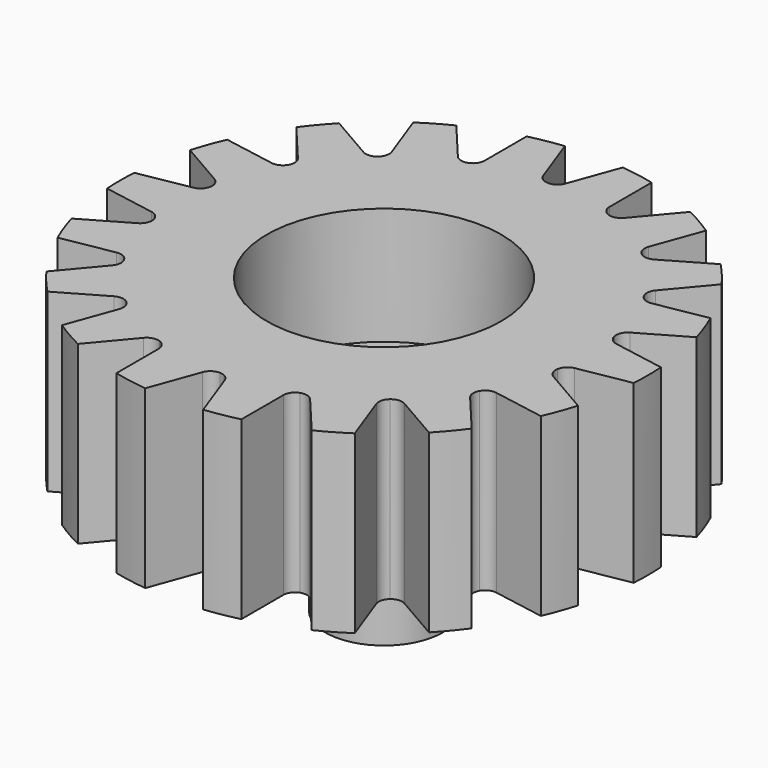
from build123d import *

# Parameters (mm, degrees)
F0_R            = 10
F0_R_2          = 5
F1_DEPTH        = 5
F2_DEPTH        = 15
F3_R            = 2
F4_DEPTH        = 8.6998377653
F0_R_3          = 22.5
F0_R_4          = 17.5
F5_DEPTH        = 5
F6_DEPTH        = 10
F8_DEPTH        = 25.0010001
F8_COPIES_COUNT = 18


# Not quite as in the source:
# - a feature of the source that left no trace in its solid (it failed there, or was rolled back) is left out
# - a pattern or mirror of a feature is missing from the dataset's text; its kind, count and spacing are read off the source's solid


with BuildPart() as f1:
    # F0 (on Top) → F1 (new body)
    with BuildSketch(Plane.XY):
        Circle(F0_R)
        Circle(F0_R_2, mode=Mode.SUBTRACT)
    extrude(amount=-F1_DEPTH)

    # F0 (on Top) → F2 (join)
    with BuildSketch(Plane.XY):
        Circle(F0_R_2)
        with BuildLine():
            ThreePointArc((2.1347076706, 1.3011622347), (2.4069450738, 0.6757332401), (2.5, 0))
            ThreePointArc((2.5, 0), (-0.6757332401, -2.4069450738), (-2.1347076706, 1.3011622347))
            ThreePointArc((-2.1347076706, 1.3011622347), (0, 2.5), (2.1347076706, 1.3011622347))
        make_face(mode=Mode.SUBTRACT)
        with BuildLine():
            Line((-2.1347076706, 1.3011622347), (2.1347076706, 1.3011622347))
            ThreePointArc((2.1347076706, 1.3011622347), (0, 2.5), (-2.1347076706, 1.3011622347))
        make_face()
    extrude(amount=-F2_DEPTH)

    # F3 (on face) → F4 (cut, through all)
    with BuildSketch(Plane.XZ.offset(-1.3011622347)):
        with Locations((0, -10)):
            Circle(F3_R)
    extrude(amount=-F4_DEPTH, mode=Mode.SUBTRACT)

    # F0 (on Top) → F5 (join)
    with BuildSketch(Plane.XY):
        Circle(F0_R_3)
        Circle(F0_R_4, mode=Mode.SUBTRACT)
        Circle(F0_R_4)
        Circle(F0_R, mode=Mode.SUBTRACT)
    extrude(amount=-F5_DEPTH)

    # F0 (on Top) → F6 (join)
    with BuildSketch(Plane.XY):
        Circle(F0_R_3)
        Circle(F0_R_4, mode=Mode.SUBTRACT)
        Circle(F0_R_4)
        Circle(F0_R, mode=Mode.SUBTRACT)
    extrude(amount=F6_DEPTH)

    # F7 (on face) → F8 (cut, through all)
    with BuildSketch(Plane.XY.offset(10)):
        with BuildLine():
            Line((0.9396926208, 18.1579798567), (2.470541887, 22.3639536483))
            ThreePointArc((2.470541887, 22.3639536483), (0, 22.5), (-2.470541887, 22.3639536483))
            Line((-2.470541887, 22.3639536483), (-0.9396926208, 18.1579798567))
            ThreePointArc((-0.9396926208, 18.1579798567), (-0.5735764364, 17.6808479557), (0, 17.5))
            ThreePointArc((0, 17.5), (0.5735764364, 17.6808479557), (0.9396926208, 18.1579798567))
        make_face()
    f8 = extrude(amount=-F8_DEPTH, mode=Mode.SUBTRACT)

    # F8_copies: F8 ×18 about axis
    f8_copies_axis = Axis((0, 0, 0), (0, 0, 1))
    for i in range(1, F8_COPIES_COUNT):
        add(f8.rotate(f8_copies_axis, i * 360 / F8_COPIES_COUNT), mode=Mode.SUBTRACT)


solid = f1.part
